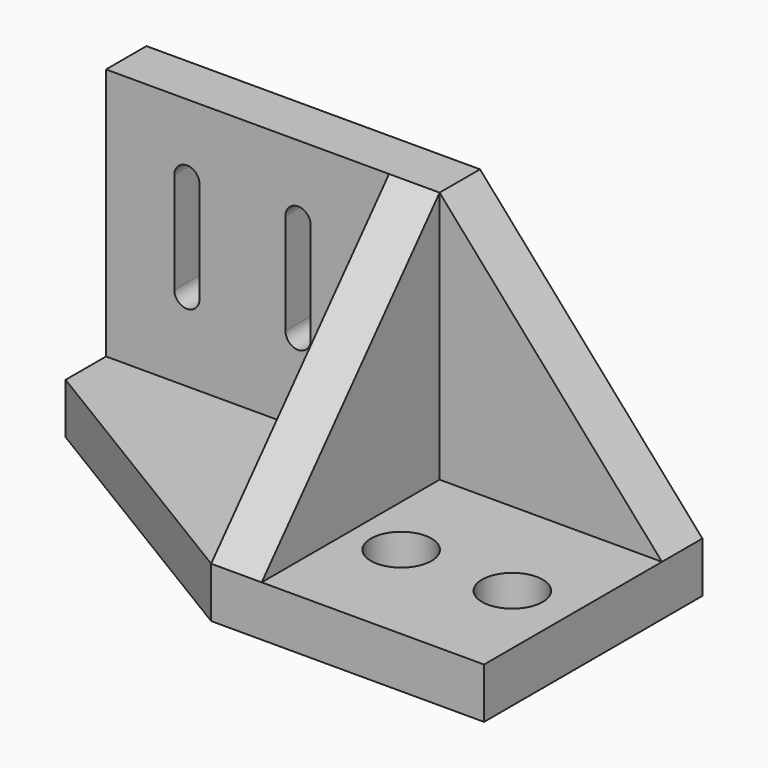
from build123d import *

# Parameters (mm, degrees)
F1_DEPTH  = 254
F3_DEPTH  = 1270
F5_DEPTH  = 701.04
F7_DEPTH  = 2278.38
F9_DEPTH  = 584.2
F10_R     = 152.4
F11_DEPTH = 1562.1


with BuildPart() as f1:
    # F0 (on Top) → F1 (new body)
    with BuildSketch(Plane.XY):
        Polygon((-1697.922529542, 314.3072188771), (-275.522529542, -549.2927811229), (1096.077470458, -549.2927811229), (1096.077470458, 822.3072188771), (-1697.922529542, 822.3072188771), align=None)
    extrude(amount=F1_DEPTH)

    # F2 (on face) → F3 (join)
    with BuildSketch(Plane.XY.offset(254)):
        Polygon((-275.522529542, 568.3072188771), (-275.522529542, -549.2927811229), (-21.522529542, -549.2927811229), (-21.522529542, 568.3072188771), (1096.077470458, 568.3072188771), (1096.077470458, 822.3072188771), (-1697.922529542, 822.3072188771), (-1697.922529542, 568.3072188771), align=None)
    extrude(amount=F3_DEPTH)

    # F4 (on face) → F5 (cut)
    with BuildSketch(Plane.XZ.offset(-568.3072188771)):
        Polygon((1096.077470458, 1524), (-21.522529542, 1524), (1096.077470458, 254), align=None)
    extrude(amount=-F5_DEPTH, mode=Mode.SUBTRACT)

    # F6 (on face) → F7 (cut)
    with BuildSketch(Plane.YZ.offset(-21.522529542)):
        Polygon((-549.2927811229, 254), (568.3072188771, 1524), (-549.2927811229, 1524), align=None)
    extrude(amount=-F7_DEPTH, mode=Mode.SUBTRACT)

    # F8 (on face) → F9 (cut)
    with BuildSketch(Plane.XZ.offset(-568.3072188771)):
        with BuildLine():
            ThreePointArc((-1355.022529542, 1168.4), (-1291.522529542, 1104.9), (-1228.022529542, 1168.4))
            ThreePointArc((-1228.022529542, 1168.4), (-1291.522529542, 1231.9), (-1355.022529542, 1168.4))
        make_face()
        with BuildLine():
            Line((-1228.022529542, 660.4), (-1228.022529542, 1168.4))
            ThreePointArc((-1228.022529542, 1168.4), (-1291.522529542, 1104.9), (-1355.022529542, 1168.4))
            Line((-1355.022529542, 1168.4), (-1355.022529542, 660.4))
            ThreePointArc((-1355.022529542, 660.4), (-1291.522529542, 723.9), (-1228.022529542, 660.4))
        make_face()
        with BuildLine():
            ThreePointArc((-1355.022529542, 660.4), (-1291.522529542, 596.9), (-1228.022529542, 660.4))
            ThreePointArc((-1228.022529542, 660.4), (-1291.522529542, 723.9), (-1355.022529542, 660.4))
        make_face()
        with BuildLine():
            ThreePointArc((-796.222529542, 1168.4), (-732.722529542, 1104.9), (-669.222529542, 1168.4))
            ThreePointArc((-669.222529542, 1168.4), (-732.722529542, 1231.9), (-796.222529542, 1168.4))
        make_face()
        with BuildLine():
            Line((-669.222529542, 660.4), (-669.222529542, 1168.4))
            ThreePointArc((-669.222529542, 1168.4), (-732.722529542, 1104.9), (-796.222529542, 1168.4))
            Line((-796.222529542, 1168.4), (-796.222529542, 660.4))
            ThreePointArc((-796.222529542, 660.4), (-732.722529542, 723.9), (-669.222529542, 660.4))
        make_face()
        with BuildLine():
            ThreePointArc((-796.222529542, 660.4), (-732.722529542, 596.9), (-669.222529542, 660.4))
            ThreePointArc((-669.222529542, 660.4), (-732.722529542, 723.9), (-796.222529542, 660.4))
        make_face()
    extrude(amount=-F9_DEPTH, mode=Mode.SUBTRACT)

    # F10 (on face) → F11 (cut)
    with BuildSketch(Plane.XY.offset(254)):
        with Locations((232.477470458, 9.5072188771)):
            Circle(F10_R)
        with Locations((791.277470458, 9.5072188771)):
            Circle(F10_R)
    extrude(amount=-F11_DEPTH, mode=Mode.SUBTRACT)


solid = f1.part
